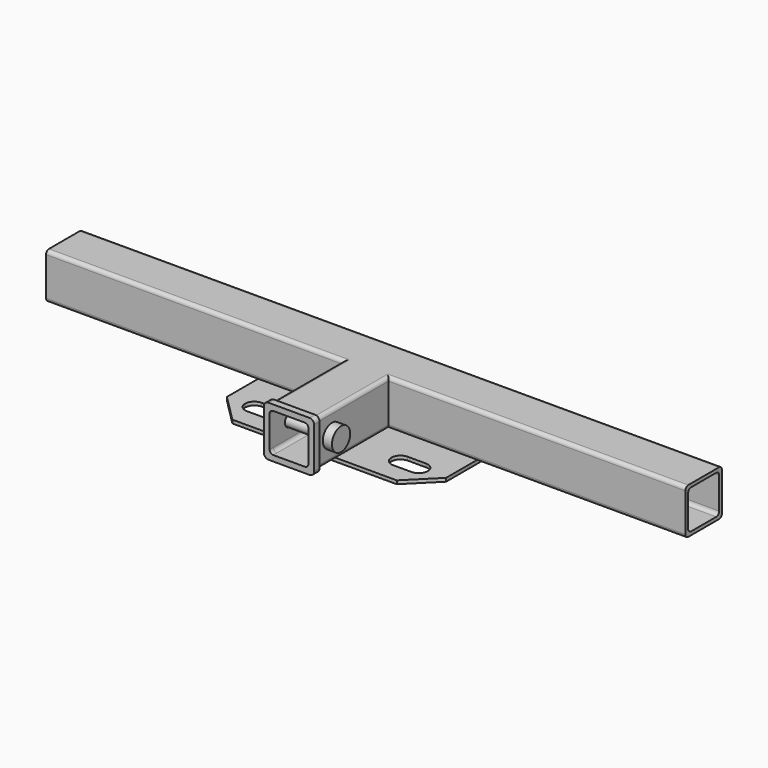
from build123d import *

# Parameters (mm, degrees)
F0_W          = 63.5
F0_H          = 63.5
F0_W_2        = 53.975
F0_H_2        = 53.975
F1_DEPTH      = 444.5
F2_W          = 63.5
F2_H          = 63.5
F2_W_2        = 53.975
F2_H_2        = 53.975
F3_DEPTH      = 127
F3_DEPTH_BACK = 63.5
F4_R          = 5.08
F7_DEPTH      = 4.7625
F9_DEPTH      = 6.35
F9_DEPTH_BACK = 3.175
F11_R         = 8.3312
F12_DEPTH     = 476.251
F13_R         = 15.875
F14_DEPTH     = 12.7
F15_R         = 7.9375
F16_DEPTH     = 76.2


with BuildPart() as f1:
    # F0 (on Right) → F1 (new body, symmetric)
    with BuildSketch(Plane.YZ):
        with Locations((-58.7375, -31.75)):
            Rectangle(F0_W, F0_H)
        with Locations((-58.7375, -31.75)):
            Rectangle(F0_W_2, F0_H_2, mode=Mode.SUBTRACT)
    extrude(amount=F1_DEPTH, both=True)

    # F2 (on face) → F3 (join, two sides)
    with BuildSketch(Plane.XZ.offset(90.4875)) as f3_sk:
        with Locations((0, -31.75)):
            Rectangle(F2_W, F2_H)
        with Locations((0, -31.75)):
            Rectangle(F2_W_2, F2_H_2, mode=Mode.SUBTRACT)
    extrude(amount=F3_DEPTH)
    extrude(f3_sk.sketch, amount=-F3_DEPTH_BACK)

    # F4
    f4_edges = [f1.edges().sort_by_distance(p)[0] for p in [
        (-238.125, -90.4875, 0),
        (238.125, -90.4875, 0),
        (0, -26.9875, 0),
        (0, -26.9875, -63.5),
        (-238.125, -90.4875, -63.5),
        (238.125, -90.4875, -63.5),
        (0, -31.75, -4.7625),
        (0, -85.725, -4.7625),
        (0, -31.75, -58.7375),
        (0, -85.725, -58.7375),
        (-31.75, -153.9875, 0),
        (31.75, -153.9875, 0),
        (31.75, -153.9875, -63.5),
        (-31.75, -153.9875, -63.5),
        (-26.9875, -153.9875, -4.7625),
        (26.9875, -153.9875, -4.7625),
        (-26.9875, -153.9875, -58.7375),
        (26.9875, -153.9875, -58.7375),
        (238.125, -85.725, -58.7375),
        (238.125, -85.725, -4.7625),
        (238.125, -31.75, -58.7375),
        (238.125, -31.75, -4.7625),
        (-238.125, -85.725, -4.7625),
        (-238.125, -85.725, -58.7375),
        (-238.125, -31.75, -58.7375),
        (-238.125, -31.75, -4.7625),
    ]]
    fillet(f4_edges, radius=F4_R)

    # F6 (on face) → F7 (join)
    with BuildSketch(Plane(origin=(0, 0, -63.5), x_dir=(1, 0, 0), z_dir=(0, 0, -1))):
        Polygon((-152.4, 26.9875), (152.4, 26.9875), (152.4, 141.2875), (114.3, 179.3875), (-114.3, 179.3875), (-152.4, 141.2875), align=None)
        with BuildLine():
            ThreePointArc((-127, 141.2875), (-123.2802561211, 150.2677561211), (-114.3, 153.9875))
            Line((-114.3, 153.9875), (-88.9, 153.9875))
            ThreePointArc((-88.9, 153.9875), (-79.9197438789, 150.2677561211), (-76.2, 141.2875))
            ThreePointArc((-76.2, 141.2875), (-79.9197438789, 132.3072438789), (-88.9, 128.5875))
            Line((-88.9, 128.5875), (-114.3, 128.5875))
            ThreePointArc((-114.3, 128.5875), (-123.2802561211, 132.3072438789), (-127, 141.2875))
        make_face(mode=Mode.SUBTRACT)
        with BuildLine():
            Line((114.3, 128.5875), (88.9, 128.5875))
            ThreePointArc((88.9, 128.5875), (79.9197438789, 132.3072438789), (76.2, 141.2875))
            ThreePointArc((76.2, 141.2875), (79.9197438789, 150.2677561211), (88.9, 153.9875))
            Line((88.9, 153.9875), (114.3, 153.9875))
            ThreePointArc((114.3, 153.9875), (123.2802561211, 150.2677561211), (127, 141.2875))
            ThreePointArc((127, 141.2875), (123.2802561211, 132.3072438789), (114.3, 128.5875))
        make_face(mode=Mode.SUBTRACT)
    extrude(amount=F7_DEPTH)

    # F8 (on face) → F9 (join, two sides)
    with BuildSketch(Plane.XZ.offset(217.4875)) as f9_sk:
        with BuildLine():
            Line((28.575, 3.175), (-28.575, 3.175))
            ThreePointArc((-28.575, 3.175), (-33.0651280605, 1.3151280605), (-34.925, -3.175))
            Line((-34.925, -3.175), (-34.925, -60.325))
            ThreePointArc((-34.925, -60.325), (-33.0651280605, -64.8151280605), (-28.575, -66.675))
            Line((-28.575, -66.675), (28.575, -66.675))
            ThreePointArc((28.575, -66.675), (33.0651280605, -64.8151280605), (34.925, -60.325))
            Line((34.925, -60.325), (34.925, -3.175))
            ThreePointArc((34.925, -3.175), (33.0651280605, 1.3151280605), (28.575, 3.175))
        make_face()
        with BuildLine():
            ThreePointArc((-26.9875, -9.8425), (-25.4996024484, -6.2503975516), (-21.9075, -4.7625))
            Line((-21.9075, -4.7625), (21.9075, -4.7625))
            ThreePointArc((21.9075, -4.7625), (25.4996024484, -6.2503975516), (26.9875, -9.8425))
            Line((26.9875, -9.8425), (26.9875, -53.6575))
            ThreePointArc((26.9875, -53.6575), (25.4996024484, -57.2496024484), (21.9075, -58.7375))
            Line((21.9075, -58.7375), (-21.9075, -58.7375))
            ThreePointArc((-21.9075, -58.7375), (-25.4996024484, -57.2496024484), (-26.9875, -53.6575))
            Line((-26.9875, -53.6575), (-26.9875, -9.8425))
        make_face(mode=Mode.SUBTRACT)
    extrude(amount=F9_DEPTH)
    extrude(f9_sk.sketch, amount=-F9_DEPTH_BACK)

    # F11 (on face) → F12 (cut, through all)
    with BuildSketch(Plane.YZ.offset(31.75)):
        with Locations((-188.9125, -31.75)):
            Circle(F11_R)
    extrude(amount=-F12_DEPTH, mode=Mode.SUBTRACT)


with BuildPart() as f14:
    # F13 (on face) → F14 (new body)
    with BuildSketch(Plane.YZ.offset(31.75)):
        with Locations((-188.9125, -31.75)):
            Circle(F13_R)
    extrude(amount=F14_DEPTH)

    # F15 (on face) → F16 (join)
    with BuildSketch(Plane(origin=(31.75, 0, 0), x_dir=(0, -1, 0), z_dir=(-1, 0, 0))):
        with Locations((188.9125, -31.75)):
            Circle(F15_R)
    extrude(amount=F16_DEPTH)


solid = Compound([f1.part, f14.part])
